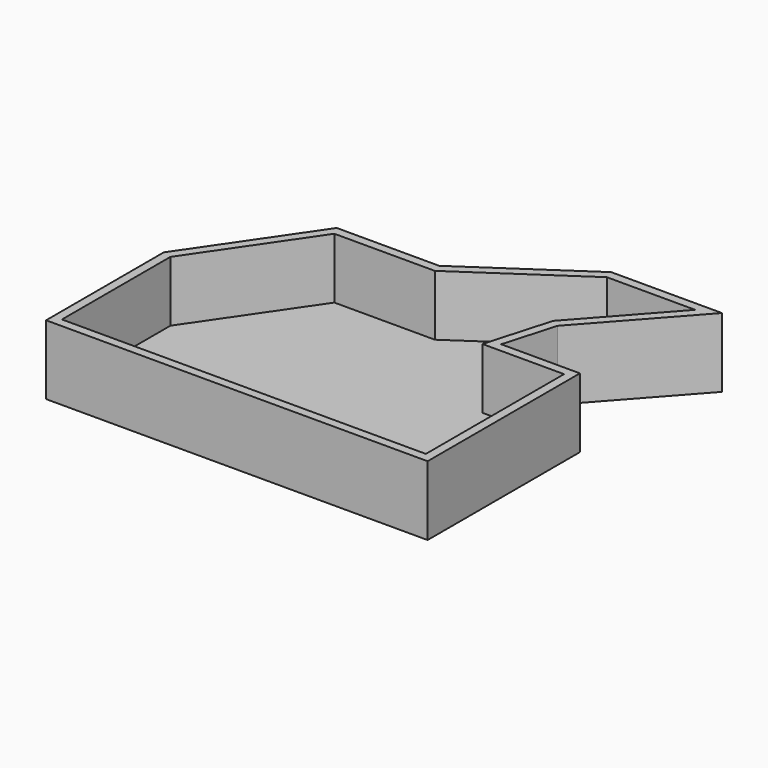
from build123d import *

# Parameters (mm, degrees)
F1_DEPTH = 20
F2_T     = -2.54


with BuildPart() as f1:
    # F0 (on Top) → F1 (new body)
    with BuildSketch(Plane.XY):
        Polygon((24.8960889876, 12.4689638615), (29.1852690279, 27.4135023355), (54.171141237, 55.3801357746), (22.2674533725, 55.3801357746), (-9.8879616708, 33.6100980639), (-39.4071526825, 33.6100980639), (-62.3756684363, 0), (-62.3756684363, -42.3790737987), (47.5712493062, -42.3790737987), (47.5712493062, 12.4689638615), align=None)
    extrude(amount=F1_DEPTH)

    # F2
    f2_openings = [f1.faces().sort_by_distance(p)[0] for p in [
        (-4.22795, -2.107401, 20),
    ]]
    offset(amount=F2_T, openings=f2_openings, kind=Kind.INTERSECTION)


solid = f1.part
